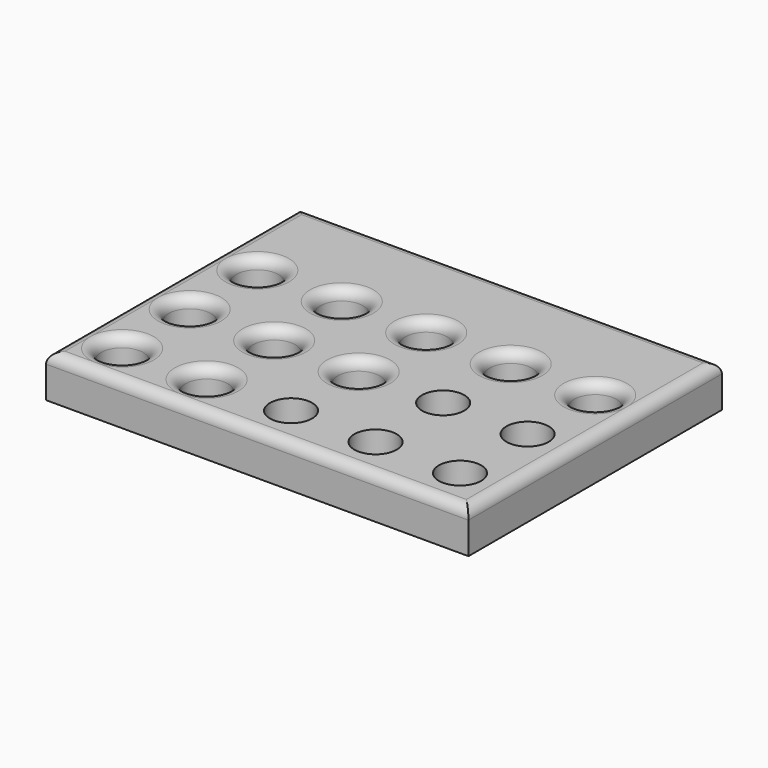
from build123d import *

# Parameters (mm, degrees)
F0_W     = 508
F0_H     = 381
F0_R     = 25.4
F1_DEPTH = 50.8
F2_R     = 12.69999


# Not quite as in the source:
# - a fillet or chamfer is up to 0.001 mm smaller than in the source, because OpenCascade refuses the exact size


with BuildPart() as f1:
    # F0 (on Top) → F1 (new body)
    with BuildSketch(Plane.XY):
        Rectangle(F0_W, F0_H)
        with Locations((-203.2, -139.7)):
            Circle(F0_R, mode=Mode.SUBTRACT)
        with Locations((-101.6, -139.7)):
            Circle(F0_R, mode=Mode.SUBTRACT)
        with Locations((0, -139.7)):
            Circle(F0_R, mode=Mode.SUBTRACT)
        with Locations((101.6, -139.7)):
            Circle(F0_R, mode=Mode.SUBTRACT)
        with Locations((203.2, -139.7)):
            Circle(F0_R, mode=Mode.SUBTRACT)
        with Locations((-203.2, -38.1)):
            Circle(F0_R, mode=Mode.SUBTRACT)
        with Locations((-101.6, -38.1)):
            Circle(F0_R, mode=Mode.SUBTRACT)
        with Locations((-203.2, 63.5)):
            Circle(F0_R, mode=Mode.SUBTRACT)
        with Locations((-101.6, 63.5)):
            Circle(F0_R, mode=Mode.SUBTRACT)
        with Locations((0, -38.1)):
            Circle(F0_R, mode=Mode.SUBTRACT)
        with Locations((0, 63.5)):
            Circle(F0_R, mode=Mode.SUBTRACT)
        with Locations((101.6, -38.1)):
            Circle(F0_R, mode=Mode.SUBTRACT)
        with Locations((203.2, -38.1)):
            Circle(F0_R, mode=Mode.SUBTRACT)
        with Locations((101.6, 63.5)):
            Circle(F0_R, mode=Mode.SUBTRACT)
        with Locations((203.2, 63.5)):
            Circle(F0_R, mode=Mode.SUBTRACT)
    extrude(amount=F1_DEPTH)

    # F2 (radius 12.7 in the source; OpenCascade refuses exactly that, so slightly less here)
    f2_edges = [f1.edges().sort_by_distance(p)[0] for p in [
        (-254, 0, 50.8),
        (0, -190.5, 50.8),
        (0, 190.5, 50.8),
        (254, 0, 50.8),
        (177.8, 63.5, 50.8),
        (76.2, 63.5, 50.8),
        (-25.4, 63.5, 50.8),
        (-127, 63.5, 50.8),
        (-228.6, 63.5, 50.8),
        (-228.6, -38.1, 50.8),
        (-228.6, -139.7, 50.8),
        (-127, -139.7, 50.8),
        (-127, -38.1, 50.8),
        (-25.4, -38.1, 50.8),
    ]]
    fillet(f2_edges, radius=F2_R)


solid = f1.part
